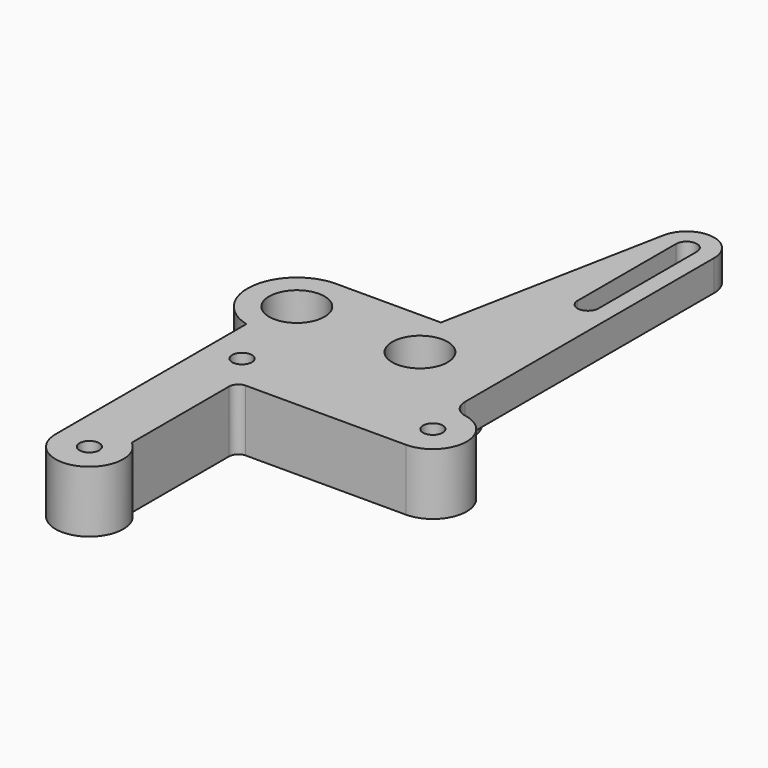
from build123d import *

# Parameters (mm, degrees)
F0_R           = 4.5
F1_DEPTH       = 5
F2_DEPTH       = 10
F4_D           = 3.2
F4_CBORE_D     = 5.6
F4_CBORE_DEPTH = 3
F5_T1_DEPTH    = 5
F6_R           = 1.5


# Not quite as in the source:
# - a fillet or chamfer that OpenCascade refuses, or shapes differently, is made with other operations: its cross-section is extruded or revolved along the edge and cut away or added
# - a feature names something its author has since deleted; it is built from what else it names


with BuildPart() as f1:
    # F0 (on Top) → F1 (new body)
    with BuildSketch(Plane.XY):
        with BuildLine():
            ThreePointArc((-12, -7.7459666924), (-5.1010205144, -6.3245553203), (-2, 0))
            ThreePointArc((-2, 0), (-4.3431457505, 5.6568542495), (-10, 8))
            ThreePointArc((-10, 8), (-17.9362375701, 1.0080343399), (-12, -7.7459666924))
        make_face()
        with Locations((-10, 0)):
            Circle(F0_R, mode=Mode.SUBTRACT)
        with BuildLine():
            ThreePointArc((-10, 8), (-4.3431457505, 5.6568542495), (-2, 0))
            ThreePointArc((-2, 0), (-5.1010205144, -6.3245553203), (-12, -7.7459666924))
            Line((-12, -7.7459666924), (-12, -15.5))
            ThreePointArc((-12, -15.5), (-6.5, -10), (-1, -15.5))
            ThreePointArc((-1, -15.5), (-1.5250628145, -17.8452078799), (-3, -19.7426406871))
            Line((-3, -19.7426406871), (-3, -21))
            Line((-3, -21), (18, -21))
            Line((18, -21), (18, -10))
            Line((18, -10), (18, 0))
            ThreePointArc((18, 0), (4.3431457505, -5.6568542495), (10, 8))
            Line((10, 8), (7, 8))
            Line((7, 8), (-10, 8))
        make_face()
        with BuildLine():
            Line((14.083025574, 44.3604283352), (7, 8))
            Line((7, 8), (10, 8))
            ThreePointArc((10, 8), (15.6568542495, 5.6568542495), (18, 0))
            Line((18, 0), (18, -10))
            Line((18, -10), (23, -10))
            Line((23, -10), (23, 43.5))
            ThreePointArc((23, 43.5), (22.2349698794, 40.9900199204), (20.2, 39.3334666688))
            Line((20.2, 39.3334666688), (20.2, 23.5))
            ThreePointArc((20.2, 23.5), (18.5, 21.8), (16.8, 23.5))
            Line((16.8, 23.5), (16.8, 39.3334666688))
            ThreePointArc((16.8, 39.3334666688), (14.5412211566, 41.3603574904), (14.083025574, 44.3604283352))
        make_face()
        with BuildLine():
            ThreePointArc((-1, -15.5), (-6.5, -10), (-12, -15.5))
            ThreePointArc((-12, -15.5), (-10.3890872965, -19.3890872965), (-6.5, -21))
            ThreePointArc((-6.5, -21), (-4.6405005753, -20.676124215), (-3, -19.7426406871))
            ThreePointArc((-3, -19.7426406871), (-1.5250628145, -17.8452078799), (-1, -15.5))
        make_face()
        with BuildLine():
            ThreePointArc((-6.5, -21), (-10.3890872965, -19.3890872965), (-12, -15.5))
            Line((-12, -15.5), (-12, -46.5))
            ThreePointArc((-12, -46.5), (-8.8452078799, -41.5250628145), (-3, -42.2573593129))
            Line((-3, -42.2573593129), (-3, -21))
            Line((-3, -21), (-6.5, -21))
        make_face()
        with BuildLine():
            ThreePointArc((23, 43.5), (18.9322123801, 47.9791955147), (14.083025574, 44.3604283352))
            ThreePointArc((14.083025574, 44.3604283352), (14.5412211566, 41.3603574904), (16.8, 39.3334666688))
            Line((16.8, 39.3334666688), (16.8, 43.5))
            ThreePointArc((16.8, 43.5), (18.5, 45.2), (20.2, 43.5))
            Line((20.2, 43.5), (20.2, 39.3334666688))
            ThreePointArc((20.2, 39.3334666688), (22.2349698794, 40.9900199204), (23, 43.5))
        make_face()
        with BuildLine():
            ThreePointArc((-3, -19.7426406871), (-4.6405005753, -20.676124215), (-6.5, -21))
            Line((-6.5, -21), (-3, -21))
            Line((-3, -21), (-3, -19.7426406871))
        make_face()
        with BuildLine():
            ThreePointArc((-3, -42.2573593129), (-8.8452078799, -41.5250628145), (-12, -46.5))
            ThreePointArc((-12, -46.5), (-6.5, -52), (-1, -46.5))
            ThreePointArc((-1, -46.5), (-1.5250628145, -44.1547921201), (-3, -42.2573593129))
        make_face()
        with BuildLine():
            Line((23, -10), (18, -10))
            Line((18, -10), (18, -21))
            Line((18, -21), (24.5, -21))
            ThreePointArc((24.5, -21), (19, -15.5), (24.5, -10))
            Line((24.5, -10), (23, -10))
        make_face()
        with BuildLine():
            ThreePointArc((30, -15.5), (28.3890872965, -11.6109127035), (24.5, -10))
            ThreePointArc((24.5, -10), (19, -15.5), (24.5, -21))
            ThreePointArc((24.5, -21), (28.3890872965, -19.3890872965), (30, -15.5))
        make_face()
        with BuildLine():
            ThreePointArc((18, 0), (15.6568542495, 5.6568542495), (10, 8))
            ThreePointArc((10, 8), (4.3431457505, -5.6568542495), (18, 0))
        make_face()
        with Locations((10, 0)):
            Circle(F0_R, mode=Mode.SUBTRACT)
    extrude(amount=-F1_DEPTH)

    # F0 (on Top) → F2 (join)
    with BuildSketch(Plane.XY):
        with BuildLine():
            ThreePointArc((30, -15.5), (28.3890872965, -11.6109127035), (24.5, -10))
            ThreePointArc((24.5, -10), (19, -15.5), (24.5, -21))
            ThreePointArc((24.5, -21), (28.3890872965, -19.3890872965), (30, -15.5))
        make_face()
        with BuildLine():
            ThreePointArc((-3, -42.2573593129), (-8.8452078799, -41.5250628145), (-12, -46.5))
            ThreePointArc((-12, -46.5), (-6.5, -52), (-1, -46.5))
            ThreePointArc((-1, -46.5), (-1.5250628145, -44.1547921201), (-3, -42.2573593129))
        make_face()
        with BuildLine():
            ThreePointArc((-12, -7.7459666924), (-5.1010205144, -6.3245553203), (-2, 0))
            ThreePointArc((-2, 0), (-4.3431457505, 5.6568542495), (-10, 8))
            ThreePointArc((-10, 8), (-17.9362375701, 1.0080343399), (-12, -7.7459666924))
        make_face()
        with Locations((-10, 0)):
            Circle(F0_R, mode=Mode.SUBTRACT)
        with BuildLine():
            ThreePointArc((-1, -15.5), (-6.5, -10), (-12, -15.5))
            ThreePointArc((-12, -15.5), (-10.3890872965, -19.3890872965), (-6.5, -21))
            ThreePointArc((-6.5, -21), (-4.6405005753, -20.676124215), (-3, -19.7426406871))
            ThreePointArc((-3, -19.7426406871), (-1.5250628145, -17.8452078799), (-1, -15.5))
        make_face()
        with BuildLine():
            ThreePointArc((-6.5, -21), (-10.3890872965, -19.3890872965), (-12, -15.5))
            Line((-12, -15.5), (-12, -46.5))
            ThreePointArc((-12, -46.5), (-8.8452078799, -41.5250628145), (-3, -42.2573593129))
            Line((-3, -42.2573593129), (-3, -21))
            Line((-3, -21), (-6.5, -21))
        make_face()
        with BuildLine():
            ThreePointArc((-3, -19.7426406871), (-4.6405005753, -20.676124215), (-6.5, -21))
            Line((-6.5, -21), (-3, -21))
            Line((-3, -21), (-3, -19.7426406871))
        make_face()
        with BuildLine():
            Line((23, -10), (18, -10))
            Line((18, -10), (18, -21))
            Line((18, -21), (24.5, -21))
            ThreePointArc((24.5, -21), (19, -15.5), (24.5, -10))
            Line((24.5, -10), (23, -10))
        make_face()
        with BuildLine():
            ThreePointArc((-10, 8), (-4.3431457505, 5.6568542495), (-2, 0))
            ThreePointArc((-2, 0), (-5.1010205144, -6.3245553203), (-12, -7.7459666924))
            Line((-12, -7.7459666924), (-12, -15.5))
            ThreePointArc((-12, -15.5), (-6.5, -10), (-1, -15.5))
            ThreePointArc((-1, -15.5), (-1.5250628145, -17.8452078799), (-3, -19.7426406871))
            Line((-3, -19.7426406871), (-3, -21))
            Line((-3, -21), (18, -21))
            Line((18, -21), (18, -10))
            Line((18, -10), (18, 0))
            ThreePointArc((18, 0), (4.3431457505, -5.6568542495), (10, 8))
            Line((10, 8), (7, 8))
            Line((7, 8), (-10, 8))
        make_face()
        with BuildLine():
            ThreePointArc((18, 0), (15.6568542495, 5.6568542495), (10, 8))
            ThreePointArc((10, 8), (4.3431457505, -5.6568542495), (18, 0))
        make_face()
        with Locations((10, 0)):
            Circle(F0_R, mode=Mode.SUBTRACT)
    extrude(amount=-F2_DEPTH)

    # F4 (through all)
    with Locations(Plane(origin=(0, 0, -10), x_dir=(1, 0, 0), z_dir=(0, 0, -1))):
        with Locations((-6.5, 46.5), (-6.5, 15.5), (24.5, 15.5)):
            CounterBoreHole(F4_D / 2, F4_CBORE_D / 2, F4_CBORE_DEPTH)

    # F5: fillet of radius 3 on 1 edges, made by hand

    # F5_s2 → F5_t1 (join)
    with BuildSketch(Plane.XY.offset(-5)):
        with BuildLine():
            ThreePointArc((25.4705882353, -10.0863174754), (23.6991050335, -9.0584665784), (23, -7.1333997347))
            Line((23, -7.1333997347), (22.7, -7.1333997347))
            Line((22.7, -7.1333997347), (22.7, -10))
            Line((22.7, -10), (23, -10.3))
            ThreePointArc((23, -10.3), (24.5, -10.3), (25.4176470588, -10.3816092494))
            Line((25.4176470588, -10.3816092494), (25.4705882353, -10.0863174754))
        make_face()
    extrude(amount=F5_T1_DEPTH)

    # F6
    f6_edges = [f1.edges().sort_by_distance(p)[0] for p in [
        (-3, -21, -5),
    ]]
    fillet(f6_edges, radius=F6_R)


solid = f1.part
